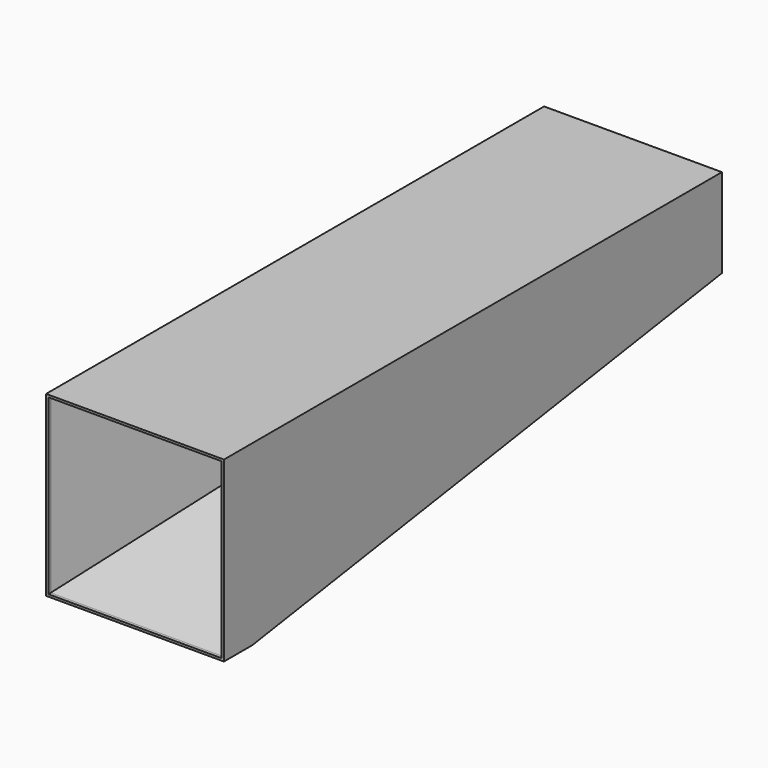
from build123d import *

# Parameters (mm, degrees)
F0_W      = 34
F0_H      = 1.332180649
F0_W_2    = 3
F0_H_2    = 30
F1_DEPTH  = 140
F3_DEPTH  = 50
F4_DEPTH  = 40
F5_T      = -0.5
F7_REACH  = 112.8020988928
F9_DEPTH  = 40
F11_DEPTH = 1000
F12_R     = 6.3171610822
F13_DEPTH = 140


# Not quite as in the source:
# - a feature names something its author has since deleted; it is built from what else it names


with BuildPart() as f1:
    # F0 (on Front) → F1 (new body)
    with BuildSketch(Plane.XZ):
        Polygon((20, 20), (17, 20), (17, 18.832180649), (17, 17.5), (17, 15), (20, 15), align=None)
        Polygon((15, 20), (-15, 20), (-17, 20), (-17, 18.832180649), (17, 18.832180649), (17, 20), align=None)
        with Locations((0, 18.1660903245)):
            Rectangle(F0_W, F0_H)
        Polygon((17, 17.5), (-17, 17.5), (-17, 15), (-17, -15), (-15, -15), (15, -15), (17, -15), (17, 15), align=None)
        Polygon((-18.5, 15), (-20, 15), (-20, -11.8550653383), (-20, -15), (-18.5, -15), (-18.5, -5.2632528394), (-18.5, -3.2632528394), (-18.5, 2.7367471606), (-18.5, 4.7367471606), align=None)
        with Locations((18.5, 0)):
            Rectangle(F0_W_2, F0_H_2)
        with BuildLine():
            Line((-15, -20), (15, -20))
            Line((15, -20), (15, -17.5))
            Line((15, -17.5), (11.391207267, -17.5))
            ThreePointArc((11.391207267, -17.5), (10.2485464886, -18.6426607784), (9.1058857102, -17.5))
            Line((9.1058857102, -17.5), (7.9234171988, -17.5))
            ThreePointArc((7.9234171988, -17.5), (5.948765669, -19.4746515298), (3.9741141393, -17.5))
            Line((3.9741141393, -17.5), (2.0740236579, -17.5))
            ThreePointArc((2.0740236579, -17.5), (0, -19.5740236579), (-2.0740236579, -17.5))
            Line((-2.0740236579, -17.5), (-3.9741141393, -17.5))
            ThreePointArc((-3.9741141393, -17.5), (-5.948765669, -19.4746515298), (-7.9234171988, -17.5))
            Line((-7.9234171988, -17.5), (-9.1058857102, -17.5))
            ThreePointArc((-9.1058857102, -17.5), (-10.2485464886, -18.6426607784), (-11.391207267, -17.5))
            Line((-11.391207267, -17.5), (-15, -17.5))
            Line((-15, -17.5), (-15, -20))
        make_face()
        Polygon((20, -20), (20, -15), (17, -15), (15, -15), (15, -17.5), (15, -20), align=None)
        Polygon((-17, -15), (-17, 15), (-18.5, 15), (-18.5, 4.7367471606), (-18.5, 2.7367471606), (-18.5, -3.2632528394), (-18.5, -5.2632528394), (-18.5, -15), align=None)
        Polygon((-15, -17.5), (-15, -15), (-16.767766953, -16.767766953), (-17.5, -17.5), (-15, -20), align=None)
        Polygon((-15, -15), (-17, -15), (-18.5, -15), (-20, -15), (-17.5, -17.5), (-16.767766953, -16.767766953), align=None)
        Polygon((-17, 18.832180649), (-17, 20), (-20, 20), (-20, 15), (-18.5, 15), (-17, 15), (-17, 17.5), align=None)
        Polygon((-17.5, -17.5), (-20, -15), (-20, -20), (-15, -20), align=None)
        with BuildLine():
            Line((3.9741141393, -17.5), (7.9234171988, -17.5))
            ThreePointArc((7.9234171988, -17.5), (5.948765669, -15.5253484702), (3.9741141393, -17.5))
        make_face()
        with BuildLine():
            ThreePointArc((3.9741141393, -17.5), (5.948765669, -19.4746515298), (7.9234171988, -17.5))
            Line((7.9234171988, -17.5), (3.9741141393, -17.5))
        make_face()
        with BuildLine():
            ThreePointArc((9.1058857102, -17.5), (10.2485464886, -18.6426607784), (11.391207267, -17.5))
            Line((11.391207267, -17.5), (9.1058857102, -17.5))
        make_face()
        with BuildLine():
            Line((9.1058857102, -17.5), (11.391207267, -17.5))
            ThreePointArc((11.391207267, -17.5), (10.2485464886, -16.3573392216), (9.1058857102, -17.5))
        make_face()
        with BuildLine():
            ThreePointArc((2.0740236579, -17.5), (0, -15.4259763421), (-2.0740236579, -17.5))
            Line((-2.0740236579, -17.5), (2.0740236579, -17.5))
        make_face()
        with BuildLine():
            Line((2.0740236579, -17.5), (-2.0740236579, -17.5))
            ThreePointArc((-2.0740236579, -17.5), (0, -19.5740236579), (2.0740236579, -17.5))
        make_face()
        with BuildLine():
            Line((-3.9741141393, -17.5), (-7.9234171988, -17.5))
            ThreePointArc((-7.9234171988, -17.5), (-5.948765669, -19.4746515298), (-3.9741141393, -17.5))
        make_face()
    extrude(amount=F1_DEPTH)


with BuildPart() as f1b:
    # F0 (on Front) → F1, piece 2 (new body)
    with BuildSketch(Plane.XZ):
        with BuildLine():
            ThreePointArc((-9.1058857102, -17.5), (-10.2485464886, -16.3573392216), (-11.391207267, -17.5))
            Line((-11.391207267, -17.5), (-9.1058857102, -17.5))
        make_face()
    extrude(amount=F1_DEPTH)


with BuildPart() as f3_tool:
    # F2 (on face) → F3 (new body)
    with BuildSketch(Plane.YZ.offset(20)):
        Polygon((0, 0), (-132.0431083441, -20), (0, -20), align=None)
    extrude(amount=-F3_DEPTH)


with BuildPart() as f1_1:
    add(f1.part)

    # F3: cut by f3_tool
    add(f3_tool.part, mode=Mode.SUBTRACT)



with BuildPart() as f1b_1:
    add(f1b.part)

    # F3: cut by f3_tool
    add(f3_tool.part, mode=Mode.SUBTRACT)


with BuildPart() as f1_2:
    add(f1_1.part)

    add(f1b_1.part)  # F4 merges F1b
    # F2 (on face) → F4 (join)
    with BuildSketch(Plane.YZ.offset(20)):
        Polygon((-133.1249161121, -12.857736984), (-132.0431083441, -20), (0, 0), (0, 7.3061197718), align=None)
        Polygon((-140, -20), (-132.0431083441, -20), (-133.1249161121, -12.857736984), (-140, -13.8990762821), align=None)
    extrude(amount=-F4_DEPTH)

    # F5
    f5_openings = [f1_2.faces().sort_by_distance(p)[0] for p in [
        (0, -140, 0),
    ]]
    offset(amount=F5_T, openings=f5_openings)

    f7_end = Plane(origin=(0, -66.021554172, -10), x_dir=(0, -0.988722747, -0.1497575692), z_dir=(0, 0.1497575692, -0.988722747))
    # F6 (on face) → F7 (join, up to a plane its end follows)
    with BuildSketch(Plane.XY.offset(20)):
        Polygon((0, -70), (-0.1507168075, -70), (0, -70.5315142328), (0.1507168075, -70), align=None)
        Polygon((0, -69.4684857672), (-0.1507168075, -70), (0, -70), (0.1507168075, -70), align=None)
        Polygon((0.1507168075, -70), (0, -70.5315142328), (19.6985663849, -140), (20, -140), align=None)
        Polygon((0, -70.5315142328), (-0.1507168075, -70), (-20, -140), (-19.6985663849, -140), align=None)
        Polygon((19.6985663849, 0), (0, -69.4684857672), (0.1507168075, -70), (20, 0), align=None)
        Polygon((-19.6985663849, 0), (-20, 0), (-0.1507168075, -70), (0, -69.4684857672), align=None)
    f7_long = extrude(amount=-F7_REACH, mode=Mode.PRIVATE)
    add(split(f7_long, bisect_by=f7_end, keep=Keep.BOTTOM, mode=Mode.PRIVATE))

    # F8 (on face) → F9 (join, through all)
    with BuildSketch(Plane.YZ.offset(20)):
        Polygon((-47.3704106226, 6.7672015175), (-46.6666666667, 6.6666666667), (-45.9831301115, 6.8619628253), (-46.6868740675, 6.9624976761), align=None)
        Polygon((-46.6868740675, 6.9624976761), (-45.9831301115, 6.8619628253), (0, 20), (-1.0556159339, 20), align=None)
        Polygon((-140, 20), (-47.3704106226, 6.7672015175), (-46.6868740675, 6.9624976761), (-137.9493903346, 20), align=None)
        Polygon((-45.9831301115, 6.8619628253), (-46.6666666667, 6.6666666667), (0, 0), (0, 0.2929442379), align=None)
        Polygon((-140, -19.6983954474), (-140, -20), (-46.6666666667, 6.6666666667), (-47.3704106226, 6.7672015175), align=None)
    extrude(amount=-F9_DEPTH)

    # F10 (on face) → F11 (cut)
    with BuildSketch(Plane(origin=(-20, 0, 0), x_dir=(0, -1, 0), z_dir=(-1, 0, 0))):
        Polygon((140, -20), (132.0431083441, -20), (132.0431083441, -21.8775942922), (142.034560442, -23.4243907034), (141.5658295155, -20), align=None)
    extrude(amount=-F11_DEPTH, mode=Mode.SUBTRACT)

    # F12 (on face) → F13 (cut, through all)
    with BuildSketch(Plane(origin=(0, 0, 0), x_dir=(-1, 0, 0), z_dir=(0, 1, 0))):
        with Locations((0, 10)):
            Circle(F12_R)
    extrude(amount=-F13_DEPTH, mode=Mode.SUBTRACT)


solid = f1_2.part
